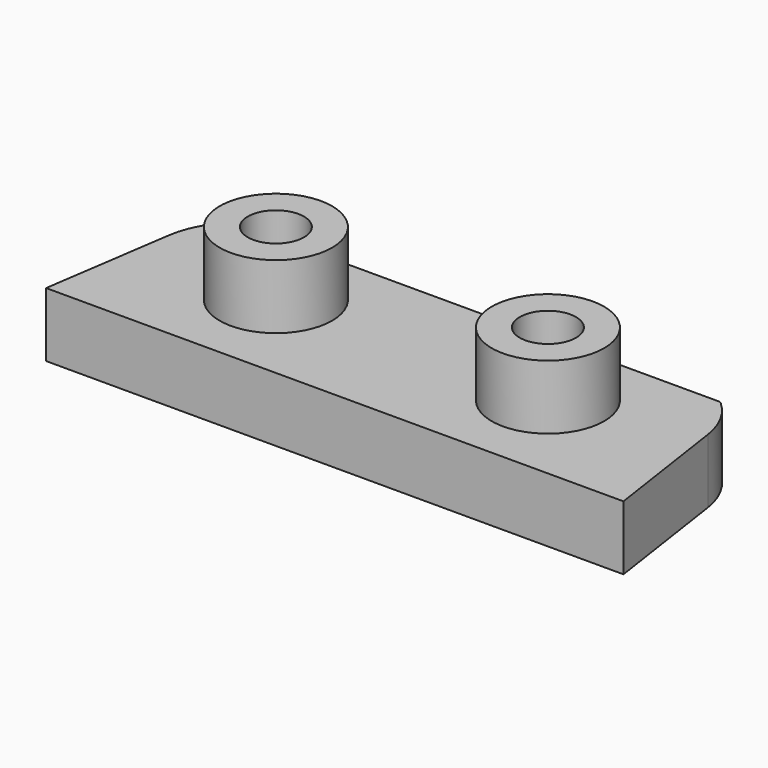
from build123d import *

# Parameters (mm, degrees)
F0_R     = 3.5
F1_DEPTH = 4
F0_R_2   = 1.75
F2_DEPTH = 4
F3_DEPTH = 8


# Not quite as in the source:
# - a feature names something its author has since deleted; it is built from what else it names


with BuildPart() as f1:
    # F0 (on Top) → F1 (new body)
    with BuildSketch(Plane.XY):
        with BuildLine():
            Line((-17.8081062952, 8.0668847322), (-19, 0))
            Line((-19, 0), (16.9281060712, 0))
            Line((16.9281060712, 0), (15.7362123664, 8.0668847322))
            ThreePointArc((15.7362123664, 8.0668847322), (15.2030202368, 9.6864800202), (14.1566041965, 11.0327326766))
            ThreePointArc((14.1566041965, 11.0327326766), (14.0697297328, 11.0864795446), (13.9693106268, 11.1052385806))
            Line((13.9693106268, 11.1052385806), (-16.0412045557, 11.1052385806))
            ThreePointArc((-16.0412045557, 11.1052385806), (-16.1416236616, 11.0864795446), (-16.2284981253, 11.0327326766))
            ThreePointArc((-16.2284981253, 11.0327326766), (-17.2749141656, 9.6864800202), (-17.8081062952, 8.0668847322))
        make_face()
        with Locations((-9.5, 6)):
            Circle(F0_R, mode=Mode.SUBTRACT)
        with Locations((7.4281060712, 6)):
            Circle(F0_R, mode=Mode.SUBTRACT)
    extrude(amount=F1_DEPTH)

    # F0 (on Top) → F3 (join)
    with BuildSketch(Plane.XY):
        with Locations((-9.5, 6)):
            Circle(F0_R)
        with Locations((-9.5, 6)):
            Circle(F0_R_2, mode=Mode.SUBTRACT)
        with Locations((7.4281060712, 6)):
            Circle(F0_R)
        with Locations((7.4281060712, 6)):
            Circle(F0_R_2, mode=Mode.SUBTRACT)
    extrude(amount=F3_DEPTH)


with BuildPart() as f2:
    # F0 (on Top) → F2 (new body)
    with BuildSketch(Plane.XY):
        with Locations((-9.5, 6)):
            Circle(F0_R_2)
    extrude(amount=F2_DEPTH)


with BuildPart() as f2b:
    # F0 (on Top) → F2, piece 2 (new body)
    with BuildSketch(Plane.XY):
        with Locations((7.4281060712, 6)):
            Circle(F0_R_2)
    extrude(amount=F2_DEPTH)


solid = Compound([f1.part, f2.part, f2b.part])
